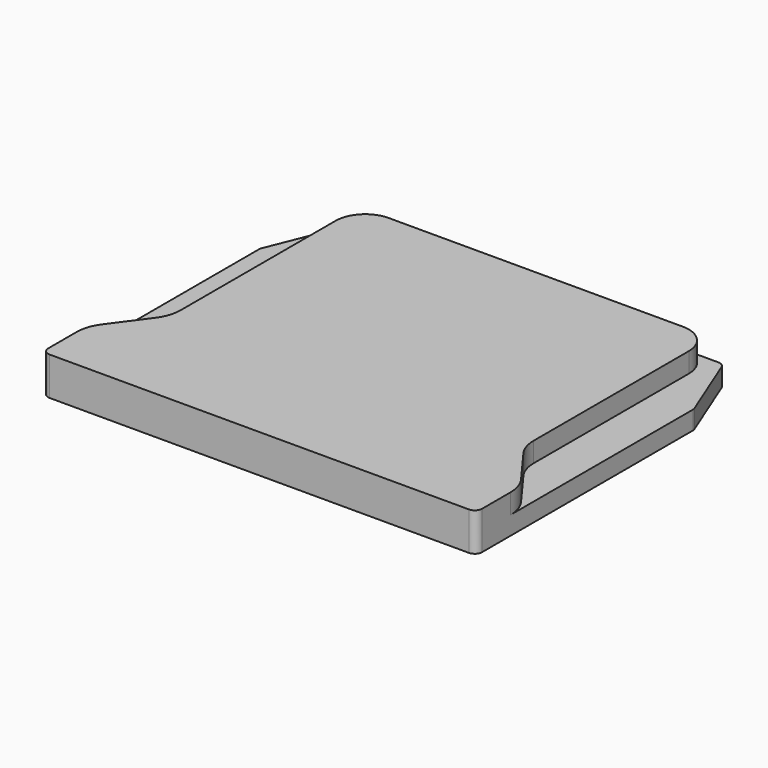
from build123d import *

# Parameters (mm, degrees)
F1_DEPTH    = 2.5
F3_DEPTH    = 2.7
F4_R        = 1
F5_R        = 5
F7_R        = 2
F8_DEPTH    = 1
F6_W        = 8
F6_H        = 15
F9_DEPTH    = 1.1
F10_SIZE2   = 1.09999
F10_SIZE    = 14.99999
F10_2_SIZE2 = 1.09999
F10_2_SIZE  = 14.99999


# Not quite as in the source:
# - a fillet or chamfer that OpenCascade refuses, or shapes differently, is made with other operations: its cross-section is extruded or revolved along the edge and cut away or added
# - two fillets or chamfers of one size are made in one step
# - a fillet or chamfer is up to 0.001 mm smaller than in the source, because OpenCascade refuses the exact size


with BuildPart() as f1:
    # F0 (on Top) → F1 (new body)
    with BuildSketch(Plane.XY):
        Polygon((55, 0), (4, 0), (0, -10), (0, -47), (59, -47), (59, -10), align=None)
    extrude(amount=F1_DEPTH)

    # F2 (on face) → F3 (join)
    with BuildSketch(Plane.XY.offset(2.5)):
        with BuildLine():
            Line((0, -39.5), (0, -47))
            Line((0, -47), (59, -47))
            Line((59, -47), (59, -39.5))
            Line((59, -39.5), (53.5, -32))
            Line((53.5, -32), (53.5, -4))
            ThreePointArc((53.5, -4), (52.3284271247, -1.1715728753), (49.5, 0))
            Line((49.5, 0), (9.5, 0))
            ThreePointArc((9.5, 0), (6.6715728753, -1.1715728753), (5.5, -4))
            Line((5.5, -4), (5.5, -32))
            Line((5.5, -32), (0, -39.5))
        make_face()
    extrude(amount=F3_DEPTH)

    # F4
    f4_edges = [f1.edges().sort_by_distance(p)[0] for p in [
        (0, -47, 2.6),
        (59, -47, 2.6),
        (4, 0, 1.25),
        (55, 0, 1.25),
        (59, -10, 1.25),
        (0, -10, 1.25),
    ]]
    fillet(f4_edges, radius=F4_R)

    # F5
    f5_edges = [f1.edges().sort_by_distance(p)[0] for p in [
        (0, -39.5, 3.85),
        (59, -39.5, 3.85),
        (53.5, -32, 3.85),
        (5.5, -32, 3.85),
    ]]
    fillet(f5_edges, radius=F5_R)

    # F7 (on face) → F8 (cut)
    with BuildSketch(Plane(origin=(0, 0, 0), x_dir=(1, 0, 0), z_dir=(0, 0, -1))):
        with Locations((19, 20)):
            Circle(F7_R)
        with Locations((40, 20)):
            Circle(F7_R)
    extrude(amount=-F8_DEPTH, mode=Mode.SUBTRACT)

    # F6 (on face) → F9 (cut)
    with BuildSketch(Plane(origin=(0, 0, 0), x_dir=(1, 0, 0), z_dir=(0, 0, -1))):
        with Locations((40, 7.5)):
            Rectangle(F6_W, F6_H)
        with Locations((19, 7.5)):
            Rectangle(F6_W, F6_H)
    extrude(amount=-F9_DEPTH, mode=Mode.SUBTRACT)

    # F10 (size 15 and 1.1 in the source; OpenCascade refuses exactly that, so slightly less here)
    f10_edges = [f1.edges().sort_by_distance(p)[0] for p in [
        (40, -15, 1.1),
    ]]
    f10_side = f1.faces().sort_by_distance((40, -7.5, 1.1))[0]
    chamfer(f10_edges, length=F10_SIZE, length2=F10_SIZE2, reference=f10_side)

    # F10#2 (size 15 and 1.1 in the source; OpenCascade refuses exactly that, so slightly less here)
    f10_2_edges = [f1.edges().sort_by_distance(p)[0] for p in [
        (19, -15, 1.1),
    ]]
    f10_2_side = f1.faces().sort_by_distance((19, -7.5, 1.1))[0]
    chamfer(f10_2_edges, length=F10_2_SIZE, length2=F10_2_SIZE2, reference=f10_2_side)

    # F12: fillet of radius 2 on 2 edges, made by hand

    # F12_s1 → F12_t2 (revolve)
    with BuildSketch(Plane.XZ.offset(20)):
        with BuildLine():
            ThreePointArc((42, 0), (41.2679491924, 0.7320508076), (40.2679491924, 1))
            Line((40.2679491924, 1), (42, 1))
            Line((42, 1), (42, 0))
        make_face()
    revolve(axis=Axis((40, -20, 1), (0, 0, -1)))

    # F12_s3 → F12_t4 (revolve)
    with BuildSketch(Plane.XZ.offset(20)):
        with BuildLine():
            ThreePointArc((21, 0), (20.2679491924, 0.7320508076), (19.2679491924, 1))
            Line((19.2679491924, 1), (21, 1))
            Line((21, 1), (21, 0))
        make_face()
    revolve(axis=Axis((19, -20, 1), (0, 0, -1)))


solid = f1.part
